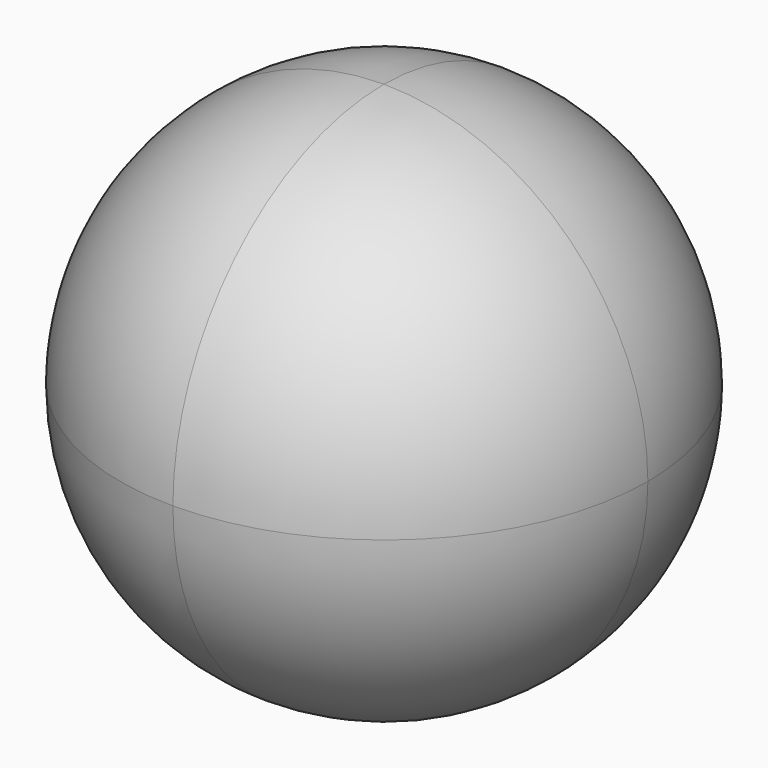
from build123d import *

# Parameters (mm, degrees)
F1_W     = 57.15
F1_H     = 57.15
F2_DEPTH = 57.15
F3_R     = 28.57499


# Not quite as in the source:
# - a fillet or chamfer is up to 0.001 mm smaller than in the source, because OpenCascade refuses the exact size


with BuildPart() as f2:
    # F1 (on Front) → F2 (new body)
    with BuildSketch(Plane.XZ):
        with Locations((1.8223590608, -2.3441536301)):
            Rectangle(F1_W, F1_H)
    extrude(amount=F2_DEPTH)

    # F3 (radius 28.575 in the source; OpenCascade refuses exactly that, so slightly less here)
    f3_edges = [f2.edges().sort_by_distance(p)[0] for p in [
        (1.822359, -57.15, 26.230846),
        (-26.752641, -57.15, -2.344154),
        (1.822359, -57.15, -30.919154),
        (30.397359, -57.15, -2.344154),
        (1.822359, 0, 26.230846),
        (-26.752641, 0, -2.344154),
        (1.822359, 0, -30.919154),
        (30.397359, 0, -2.344154),
        (-26.752641, -28.575, -30.919154),
        (30.397359, -28.575, -30.919154),
        (30.397359, -28.575, 26.230846),
        (-26.752641, -28.575, 26.230846),
    ]]
    fillet(f3_edges, radius=F3_R)


solid = f2.part
